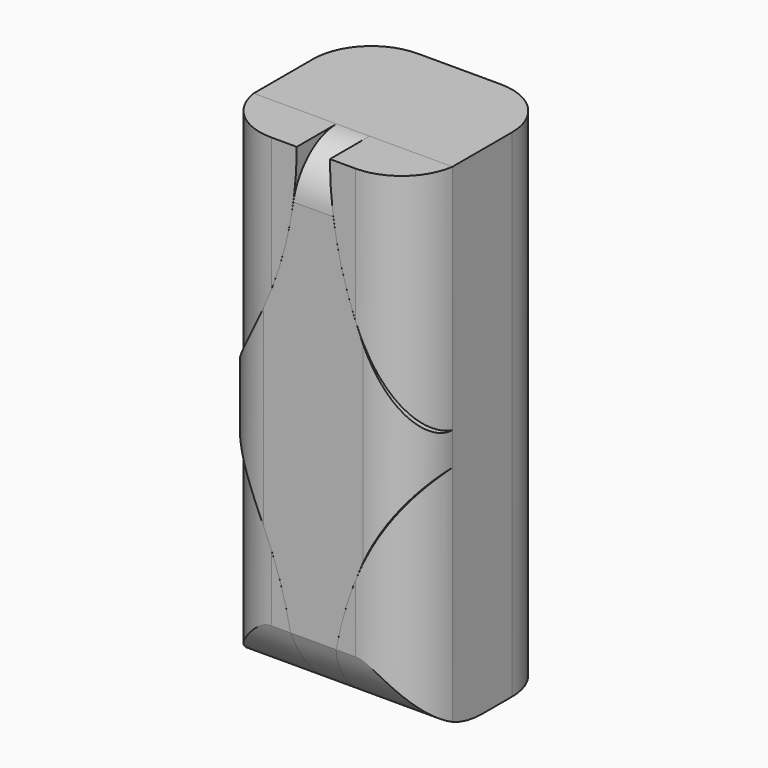
from build123d import *

# Parameters (mm, degrees)
F2_W           = 304.8
F2_H           = 203.2
F3_DEPTH       = 762
F7_DEPTH       = 76.2
F8_F1_R        = 88.9
F8_F2_R        = 88.9
F8_2_T1_DEPTH  = 795.5409051225
F8_3_T1_DEPTH  = 795.5409051225
F8_4_T1_DEPTH  = 795.5409051225
F8_5_T1_DEPTH  = 795.5409051225
F10_DEPTH      = 76.2
F11_R          = 76.19999
F12_R          = 76.19999
F14_DEPTH      = 152.4010001
F14_DEPTH_BACK = 152.4010001


# Not quite as in the source:
# - a fillet or chamfer that OpenCascade refuses, or shapes differently, is made with other operations: its cross-section is extruded or revolved along the edge and cut away or added
# - a fillet or chamfer is up to 0.001 mm smaller than in the source, because OpenCascade refuses the exact size


with BuildPart() as f3:
    # F2 (on plane+point) → F3 (new body, through all)
    with BuildSketch(Plane.XY.offset(-381)):
        with Locations((0, 101.6)):
            Rectangle(F2_W, F2_H)
    extrude(amount=F3_DEPTH)

    # F8: fillet of radius 88.9 on 2 edges, made by hand

    # F8_f1
    f8_f1_edges = [f3.edges().sort_by_distance(p)[0] for p in [
        (-152.4, 203.2, 0),
    ]]
    fillet(f8_f1_edges, radius=F8_F1_R)

    # F8_f2
    f8_f2_edges = [f3.edges().sort_by_distance(p)[0] for p in [
        (152.4, 203.2, 0),
    ]]
    fillet(f8_f2_edges, radius=F8_F2_R)


with BuildPart() as f7:
    # F6 (on plane+point) → F7 (new body, through all)
    with BuildSketch(Plane.XZ.offset(76.2)):
        with BuildLine():
            Line((-25.4, 381), (-152.4, 381))
            Line((-152.4, 381), (-152.4, 25.4))
            ThreePointArc((-152.4, 25.4), (-58.1025953454, 192.2009269091), (-25.4, 381))
        make_face()
    extrude(amount=-F7_DEPTH)

    # F8#2: fillet of radius 88.9 on 1 edges, made by hand

    # F8_2_s2 → F8_2_t1 (cut)
    with BuildSketch(Plane.XY.offset(-194.5704525613)):
        with BuildLine():
            ThreePointArc((-152.4, 0), (-122.6105303014, -54.502083301), (-64.4118189755, -76.2))
            Line((-64.4118189755, -76.2), (-152.4, -76.2))
            Line((-152.4, -76.2), (-152.4, 0))
        make_face()
    extrude(amount=F8_2_T1_DEPTH, mode=Mode.SUBTRACT)


with BuildPart() as f7b:
    # F6 (on plane+point) → F7, piece 2 (new body, through all)
    with BuildSketch(Plane.XZ.offset(76.2)):
        with BuildLine():
            Line((152.4, 25.4), (152.4, 381))
            Line((152.4, 381), (25.4, 381))
            ThreePointArc((25.4, 381), (58.1025953454, 192.2009269091), (152.4, 25.4))
        make_face()
    extrude(amount=-F7_DEPTH)

    # F8#3: fillet of radius 88.9 on 1 edges, made by hand

    # F8_3_s2 → F8_3_t1 (cut)
    with BuildSketch(Plane.XY.offset(-194.5704525613)):
        with BuildLine():
            ThreePointArc((152.4, 0), (122.6105303014, -54.502083301), (64.4118189755, -76.2))
            Line((64.4118189755, -76.2), (152.4, -76.2))
            Line((152.4, -76.2), (152.4, 0))
        make_face()
    extrude(amount=F8_3_T1_DEPTH, mode=Mode.SUBTRACT)


with BuildPart() as f7c:
    # F6 (on plane+point) → F7, piece 3 (new body, through all)
    with BuildSketch(Plane.XZ.offset(76.2)):
        with BuildLine():
            Line((25.4, -381), (152.4, -381))
            Line((152.4, -381), (152.4, -25.4))
            ThreePointArc((152.4, -25.4), (58.1025953454, -192.2009269091), (25.4, -381))
        make_face()
    extrude(amount=-F7_DEPTH)

    # F8#4: fillet of radius 88.9 on 1 edges, made by hand

    # F8_4_s2 → F8_4_t1 (cut)
    with BuildSketch(Plane.XY.offset(-600.9704525612)):
        with BuildLine():
            ThreePointArc((152.4, 0), (122.6105303014, -54.502083301), (64.4118189755, -76.2))
            Line((64.4118189755, -76.2), (152.4, -76.2))
            Line((152.4, -76.2), (152.4, 0))
        make_face()
    extrude(amount=F8_4_T1_DEPTH, mode=Mode.SUBTRACT)


with BuildPart() as f7d:
    # F6 (on plane+point) → F7, piece 4 (new body, through all)
    with BuildSketch(Plane.XZ.offset(76.2)):
        with BuildLine():
            Line((-152.4, -381), (-25.4, -381))
            ThreePointArc((-25.4, -381), (-58.1025953454, -192.2009269091), (-152.4, -25.4))
            Line((-152.4, -25.4), (-152.4, -381))
        make_face()
    extrude(amount=-F7_DEPTH)

    # F8#5: fillet of radius 88.9 on 1 edges, made by hand

    # F8_5_s2 → F8_5_t1 (cut)
    with BuildSketch(Plane.XY.offset(-600.9704525612)):
        with BuildLine():
            ThreePointArc((-152.4, 0), (-122.6105303014, -54.502083301), (-64.4118189755, -76.2))
            Line((-64.4118189755, -76.2), (-152.4, -76.2))
            Line((-152.4, -76.2), (-152.4, 0))
        make_face()
    extrude(amount=F8_5_T1_DEPTH, mode=Mode.SUBTRACT)


with BuildPart() as f10:
    # F9 (on face) → F10 (new body, through all)
    with BuildSketch(Plane.XZ):
        with BuildLine():
            ThreePointArc((-64.4118189755, 175.3890399136), (-102.5626769357, 96.9667001384), (-152.4, 25.4))
            Line((-152.4, 25.4), (-152.4, -25.4))
            ThreePointArc((-152.4, -25.4), (-102.5626769357, -96.9667001384), (-64.4118189755, -175.3890399136))
            ThreePointArc((-64.4118189755, -175.3890399136), (-35.2391855236, -276.3603935794), (-25.4, -381))
            Line((-25.4, -381), (25.4, -381))
            ThreePointArc((25.4, -381), (35.2391855236, -276.3603935794), (64.4118189755, -175.3890399136))
            ThreePointArc((64.4118189755, -175.3890399136), (102.5626769357, -96.9667001384), (152.4, -25.4))
            Line((152.4, -25.4), (152.4, 25.4))
            ThreePointArc((152.4, 25.4), (102.5626769357, 96.9667001384), (64.4118189755, 175.3890399136))
            ThreePointArc((64.4118189755, 175.3890399136), (35.2391855236, 276.3603935794), (25.4, 381))
            Line((25.4, 381), (-25.4, 381))
            ThreePointArc((-25.4, 381), (-35.2391855236, 276.3603935794), (-64.4118189755, 175.3890399136))
        make_face()
    extrude(amount=F10_DEPTH)

    # F11 (radius 76.2 in the source; OpenCascade refuses exactly that, so slightly less here)
    f11_edges = [f10.edges().sort_by_distance(p)[0] for p in [
        (-152.4, -76.2, 0),
        (152.4, -76.2, 0),
    ]]
    fillet(f11_edges, radius=F11_R)

    # F12 (radius 76.2 in the source; OpenCascade refuses exactly that, so slightly less here)
    f12_edges = [f10.edges().sort_by_distance(p)[0] for p in [
        (0, -76.2, 381),
    ]]
    fillet(f12_edges, radius=F12_R)


with BuildPart() as f14_tool:
    # F13 (on Right) → F14 (new body, two sides)
    with BuildSketch(Plane.YZ) as f14_sk:
        with BuildLine():
            ThreePointArc((57.15, -381), (-27.0390569298, -352.3149155996), (-76.2, -278.1945199568))
            Line((-76.2, -278.1945199568), (-76.2, -381))
            Line((-76.2, -381), (57.15, -381))
        make_face()
    extrude(amount=-F14_DEPTH)
    extrude(f14_sk.sketch, amount=F14_DEPTH_BACK)


with BuildPart() as f3_1:
    add(f3.part)

    # F14: cut by f14_tool
    add(f14_tool.part, mode=Mode.SUBTRACT)


with BuildPart() as f7c_1:
    add(f7c.part)

    # F14: cut by f14_tool
    add(f14_tool.part, mode=Mode.SUBTRACT)


with BuildPart() as f7d_1:
    add(f7d.part)

    # F14: cut by f14_tool
    add(f14_tool.part, mode=Mode.SUBTRACT)


with BuildPart() as f10_1:
    add(f10.part)

    # F14: cut by f14_tool
    add(f14_tool.part, mode=Mode.SUBTRACT)


solid = Compound([f7.part, f7b.part, f3_1.part, f7c_1.part, f7d_1.part, f10_1.part])
